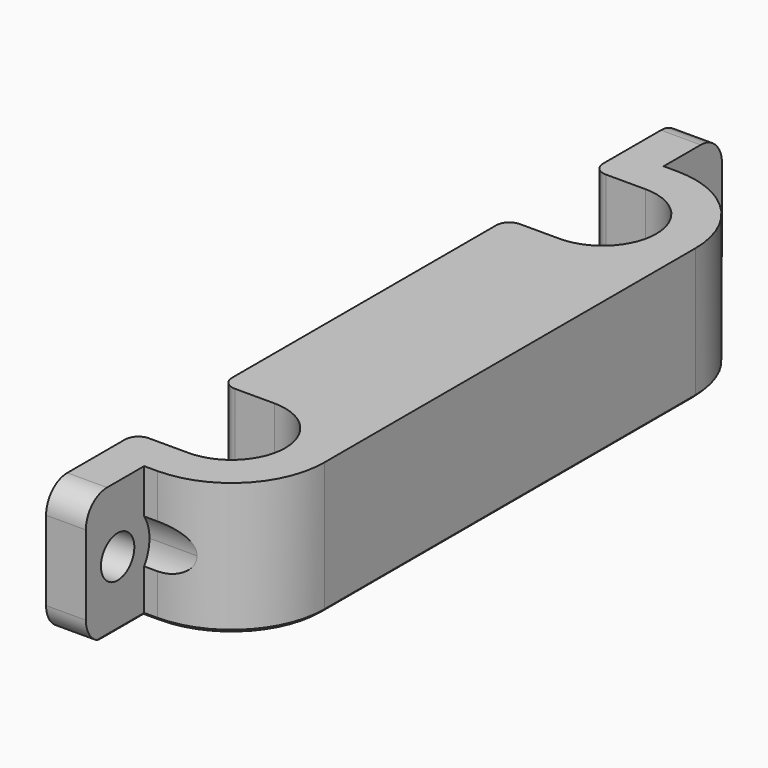
from build123d import *

# Parameters (mm, degrees)
F1_DEPTH     = 5
F2_R         = 1
F3_R         = 1.575
F4_DEPTH     = 3
F3_R_2       = 3
F5_DEPTH     = 8.001
F6_R         = 2
F7_T1_DEPTH  = 6.5429652699
F7_T3_DEPTH  = 3
F7_T5_DEPTH  = 35
F7_T7_DEPTH  = 24.9
F7_T9_DEPTH  = 6.5429652699
F7_T12_ANGLE = 90
F7_T16_DEPTH = 5.2358860169
F7_T21_DEPTH = 1.642920747
F7_T24_ANGLE = 180
F7_T26_ANGLE = 90
F7_T28_ANGLE = 90
F7_T30_ANGLE = 90
F7_T34_DEPTH = 1.642920747
F7_T37_ANGLE = 90
F7_T41_DEPTH = 5.2358860169
F7_T44_ANGLE = 180
F7_T46_ANGLE = 90


# Not quite as in the source:
# - a fillet or chamfer that OpenCascade refuses, or shapes differently, is made with other operations: its cross-section is extruded or revolved along the edge and cut away or added


with BuildPart() as f1:
    # F0 (on Top) → F1 (new body, symmetric)
    with BuildSketch(Plane.XY):
        with BuildLine():
            Line((-4, 21.55), (0, 21.55))
            ThreePointArc((0, 21.55), (4.05, 17.5), (0, 13.45))
            Line((0, 13.45), (-4, 13.45))
            Line((-4, 13.45), (-4, 0))
            Line((-4, 0), (-4, -13.45))
            Line((-4, -13.45), (0, -13.45))
            ThreePointArc((0, -13.45), (4.05, -17.5), (0, -21.55))
            Line((0, -21.55), (-4, -21.55))
            Line((-4, -21.55), (-4, -30))
            Line((-4, -30), (-1, -30))
            Line((-1, -30), (-1, -24.5))
            Line((-1, -24.5), (0, -24.5))
            ThreePointArc((0, -24.5), (4.9497474683, -22.4497474683), (7, -17.5))
            Line((7, -17.5), (7, 0))
            Line((7, 0), (7, 17.5))
            ThreePointArc((7, 17.5), (4.9497474683, 22.4497474683), (0, 24.5))
            Line((0, 24.5), (-1, 24.5))
            Line((-1, 24.5), (-1, 30))
            Line((-1, 30), (-4, 30))
            Line((-4, 30), (-4, 21.55))
        make_face()
    extrude(amount=F1_DEPTH, both=True)

    # F2
    f2_edges = [f1.edges().sort_by_distance(p)[0] for p in [
        (-4, 21.55, 0),
        (-4, 13.45, 0),
        (-4, -21.55, 0),
        (-4, -13.45, 0),
    ]]
    fillet(f2_edges, radius=F2_R)

    # F3 (on face) → F4 (cut, through all)
    with BuildSketch(Plane.YZ.offset(-1)):
        with Locations((27, 0)):
            Circle(F3_R)
        with Locations((-27, 0)):
            Circle(F3_R)
    extrude(amount=-F4_DEPTH, mode=Mode.SUBTRACT)

    # F3 (on face) → F5 (cut, through all)
    with BuildSketch(Plane.YZ.offset(-1)):
        with Locations((27, 0)):
            Circle(F3_R_2)
        with Locations((27, 0)):
            Circle(F3_R, mode=Mode.SUBTRACT)
        with BuildLine():
            ThreePointArc((-24.5, -1.6583123952), (-24.1277186767, -0.8660254038), (-24, 0))
            ThreePointArc((-24, 0), (-24.1277186767, 0.8660254038), (-24.5, 1.6583123952))
            Line((-24.5, 1.6583123952), (-24.5, -1.6583123952))
        make_face()
        with BuildLine():
            Line((-24.5, -1.6583123952), (-24.5, 1.6583123952))
            ThreePointArc((-24.5, 1.6583123952), (-27.8660254038, 2.8722813233), (-30, 0))
            ThreePointArc((-30, 0), (-27.8660254038, -2.8722813233), (-24.5, -1.6583123952))
        make_face()
        with Locations((-27, 0)):
            Circle(F3_R, mode=Mode.SUBTRACT)
    extrude(amount=F5_DEPTH, mode=Mode.SUBTRACT)

    # F6
    f6_edges = [f1.edges().sort_by_distance(p)[0] for p in [
        (-2.5, 30, -5),
        (-2.5, 30, 5),
        (-2.5, -30, -5),
        (-2.5, -30, 5),
    ]]
    fillet(f6_edges, radius=F6_R)

    # F7: chamfer of 0.25 on 22 edges, made by hand

    # F7_s2 → F7_t1 (cut)
    with BuildSketch(Plane.XZ.offset(-29.0929652699)):
        Polygon((-3.75, -5), (-4, -4.75), (-4, -5), align=None)
    extrude(amount=F7_T1_DEPTH, mode=Mode.SUBTRACT)

    # F7_s4 → F7_t3 (cut)
    with BuildSketch(Plane.YZ.offset(-3)):
        Polygon((21.8, -5), (21.55, -4.75), (21.55, -5), align=None)
        Polygon((13.2, -5), (13.45, -4.75), (13.45, -5), align=None)
        Polygon((-13.2, -5), (-13.45, -4.75), (-13.45, -5), align=None)
        Polygon((-21.8, -5), (-21.55, -4.75), (-21.55, -5), align=None)
    extrude(amount=F7_T3_DEPTH, mode=Mode.SUBTRACT)

    # F7_s6 → F7_t5 (cut)
    with BuildSketch(Plane.XZ.offset(-17.5)):
        Polygon((6.75, -5), (7, -4.75), (7, -5), align=None)
    extrude(amount=F7_T5_DEPTH, mode=Mode.SUBTRACT)

    # F7_s8 → F7_t7 (cut)
    with BuildSketch(Plane.XZ.offset(-12.45)):
        Polygon((-3.75, -5), (-4, -4.75), (-4, -5), align=None)
    extrude(amount=F7_T7_DEPTH, mode=Mode.SUBTRACT)

    # F7_s10 → F7_t9 (cut)
    with BuildSketch(Plane.XZ.offset(22.55)):
        Polygon((-4, -4.75), (-3.75, -5), (-4, -5), align=None)
    extrude(amount=F7_T9_DEPTH, mode=Mode.SUBTRACT)

    # F7_s11 → F7_t12 (revolve, cut)
    with BuildSketch(Plane.YZ.offset(-3)):
        Polygon((21.8, -5), (21.55, -4.75), (21.55, -5), align=None)
    revolve(axis=Axis((-3, 22.55, -5), (0, 0, -1)), revolution_arc=F7_T12_ANGLE, mode=Mode.SUBTRACT)


with BuildPart() as f7_tool14:
    # F7_s15 → F7_t16 (new body)
    with BuildSketch(Plane.XZ.offset(-23.857079253)):
        Polygon((-1.25, -5), (-1, -4.75), (-1, -5), align=None)
    extrude(amount=-F7_T16_DEPTH)

    split(bisect_by=Plane(origin=(0, 14.625, -14.625), x_dir=(1, 0, 0), z_dir=(0, 0.7071067812, -0.7071067812)), keep=Keep.TOP)


with BuildPart() as f1_1:
    add(f1.part)

    # F7_t13: cut F7_tool14
    add(f7_tool14.part, mode=Mode.SUBTRACT)


with BuildPart() as f7_tool19:
    # F7_s20 → F7_t21 (new body)
    with BuildSketch(Plane.YZ):
        Polygon((24.25, -5), (24.5, -4.75), (24.5, -5), align=None)
    extrude(amount=-F7_T21_DEPTH)

    split(bisect_by=Plane(origin=(1.875, 0, -1.875), x_dir=(0, 1, 0), z_dir=(0.7071067812, 0, -0.7071067812)), keep=Keep.TOP)


with BuildPart() as f1_2:
    add(f1_1.part)

    # F7_t18: cut F7_tool19
    add(f7_tool19.part, mode=Mode.SUBTRACT)

    # F7_s23 → F7_t24 (revolve, cut)
    with BuildSketch(Plane.YZ):
        Polygon((21.8, -5), (21.55, -4.75), (21.55, -5), align=None)
    revolve(axis=Axis((0, 17.5, -5), (0, 0, -1)), revolution_arc=F7_T24_ANGLE, mode=Mode.SUBTRACT)

    # F7_s25 → F7_t26 (revolve, cut)
    with BuildSketch(Plane.XZ.offset(-17.5)):
        Polygon((6.75, -5), (7, -4.75), (7, -5), align=None)
    revolve(axis=Axis((0, 17.5, -5), (0, 0, 1)), revolution_arc=F7_T26_ANGLE, mode=Mode.SUBTRACT)

    # F7_s27 → F7_t28 (revolve, cut)
    with BuildSketch(Plane.XZ.offset(-12.45)):
        Polygon((-3.75, -5), (-4, -4.75), (-4, -5), align=None)
    revolve(axis=Axis((-3, 12.45, -5), (0, 0, -1)), revolution_arc=F7_T28_ANGLE, mode=Mode.SUBTRACT)

    # F7_s29 → F7_t30 (revolve, cut)
    with BuildSketch(Plane.YZ):
        Polygon((-24.25, -5), (-24.5, -4.75), (-24.5, -5), align=None)
    revolve(axis=Axis((0, -17.5, -5), (0, 0, 1)), revolution_arc=F7_T30_ANGLE, mode=Mode.SUBTRACT)


with BuildPart() as f7_tool32:
    # F7_s33 → F7_t34 (new body)
    with BuildSketch(Plane.YZ.offset(-1.642920747)):
        Polygon((-24.25, -5), (-24.5, -4.75), (-24.5, -5), align=None)
    extrude(amount=F7_T34_DEPTH)

    split(bisect_by=Plane(origin=(1.875, 0, -1.875), x_dir=(0, 1, 0), z_dir=(0.7071067812, 0, -0.7071067812)), keep=Keep.TOP)


with BuildPart() as f1_3:
    add(f1_2.part)

    # F7_t31: cut F7_tool32
    add(f7_tool32.part, mode=Mode.SUBTRACT)

    # F7_s36 → F7_t37 (revolve, cut)
    with BuildSketch(Plane.YZ.offset(-3)):
        Polygon((-13.2, -5), (-13.45, -4.75), (-13.45, -5), align=None)
    revolve(axis=Axis((-3, -12.45, -5), (0, 0, -1)), revolution_arc=F7_T37_ANGLE, mode=Mode.SUBTRACT)


with BuildPart() as f7_tool39:
    # F7_s40 → F7_t41 (new body)
    with BuildSketch(Plane.XZ.offset(29.0929652699)):
        Polygon((-1.25, -5), (-1, -4.75), (-1, -5), align=None)
    extrude(amount=-F7_T41_DEPTH)

    split(bisect_by=Plane(origin=(0, -14.625, -14.625), x_dir=(1, 0, 0), z_dir=(0, -0.7071067812, -0.7071067812)), keep=Keep.TOP)


with BuildPart() as f1_4:
    add(f1_3.part)

    # F7_t38: cut F7_tool39
    add(f7_tool39.part, mode=Mode.SUBTRACT)

    # F7_s43 → F7_t44 (revolve, cut)
    with BuildSketch(Plane.YZ):
        Polygon((-13.2, -5), (-13.45, -4.75), (-13.45, -5), align=None)
    revolve(axis=Axis((0, -17.5, -5), (0, 0, -1)), revolution_arc=F7_T44_ANGLE, mode=Mode.SUBTRACT)

    # F7_s45 → F7_t46 (revolve, cut)
    with BuildSketch(Plane.XZ.offset(22.55)):
        Polygon((-3.75, -5), (-4, -4.75), (-4, -5), align=None)
    revolve(axis=Axis((-3, -22.55, -5), (0, 0, -1)), revolution_arc=F7_T46_ANGLE, mode=Mode.SUBTRACT)


solid = f1_4.part
